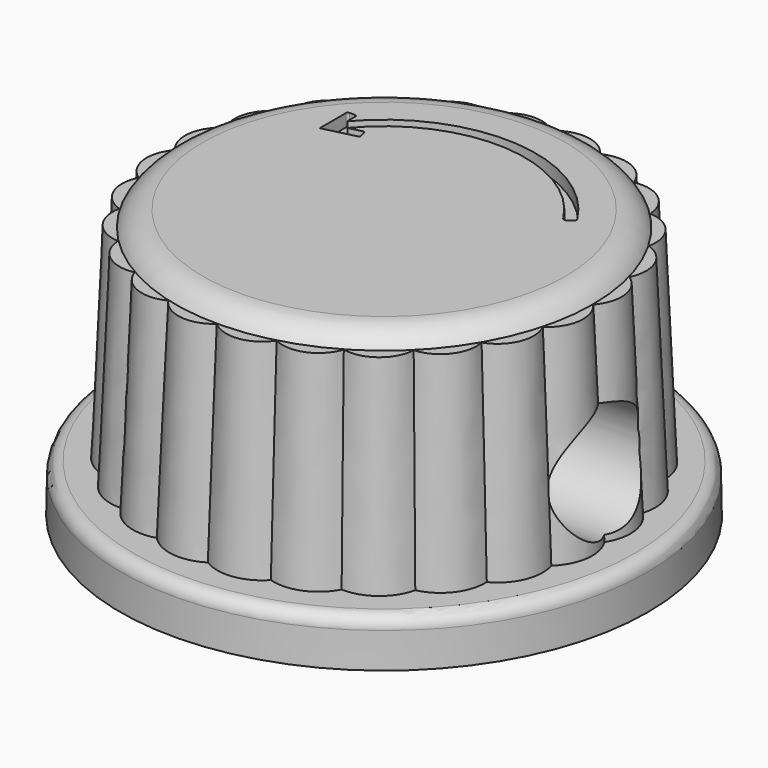
from build123d import *

# Parameters (mm, degrees)
F0_R                   = 8.35
F1_DEPTH               = 1.5
F1_TAPER               = 1
F2_R                   = 6.9
F3_DEPTH               = 6.5
F3_TAPER               = 2.5
F4_R                   = 6.6019829431
F5_DEPTH               = 0.5
F7_DEPTH               = 6.5
DRAFT_F7_DRAFTED_ANGLE = -2.5
F9_R                   = 0.4
F10_R                  = 3.9
F11_DEPTH              = 6.8
F12_R                  = 1.8
F13_DEPTH              = 25
F15_DEPTH              = 0.4


# Not quite as in the source:
# - a fillet or chamfer that OpenCascade refuses, or shapes differently, is made with other operations: its cross-section is extruded or revolved along the edge and cut away or added
# - an extrude with a draft is written as a straight extrude whose walls are then drafted


with BuildPart() as f1:
    # F0 (on Top) → F1 (new body)
    with BuildSketch(Plane.XY):
        Circle(F0_R)
    extrude(amount=F1_DEPTH, taper=F1_TAPER)

    # F2 (on face) → F3 (join)
    with BuildSketch(Plane.XY.offset(1.5)):
        Circle(F2_R)
    extrude(amount=F3_DEPTH, taper=F3_TAPER)

    # F4 (on face) → F5 (join)
    with BuildSketch(Plane.XY.offset(8)):
        Circle(F4_R)
    extrude(amount=F5_DEPTH)


with BuildPart() as f7_drafted:
    # F6 (on face) → F7 (new body, through all)
    with BuildSketch(Plane.XY.offset(8)):
        with BuildLine():
            ThreePointArc((6.3907621911, -1.7123995681), (6.8957390773, -0.9078412722), (6.6162038711, 0))
            ThreePointArc((6.6162038711, 0), (6.8957390773, 0.9078412722), (6.3907621911, 1.7123995681))
            ThreePointArc((6.3907621911, 1.7123995681), (6.4258058549, 2.6616559343), (5.729800629, 3.3081019355))
            ThreePointArc((5.729800629, 3.3081019355), (5.5179645827, 4.234083143), (4.678362623, 4.678362623))
            ThreePointArc((4.678362623, 4.678362623), (4.234083143, 5.5179645827), (3.3081019355, 5.729800629))
            ThreePointArc((3.3081019355, 5.729800629), (2.6616559343, 6.4258058549), (1.7123995681, 6.3907621911))
            ThreePointArc((1.7123995681, 6.3907621911), (0.9078412722, 6.8957390773), (0, 6.6162038711))
            ThreePointArc((0, 6.6162038711), (-0.9078412722, 6.8957390773), (-1.7123995681, 6.3907621911))
            ThreePointArc((-1.7123995681, 6.3907621911), (-2.6616559343, 6.4258058549), (-3.3081019355, 5.729800629))
            ThreePointArc((-3.3081019355, 5.729800629), (-4.234083143, 5.5179645827), (-4.678362623, 4.678362623))
            ThreePointArc((-4.678362623, 4.678362623), (-5.5179645827, 4.234083143), (-5.729800629, 3.3081019355))
            ThreePointArc((-5.729800629, 3.3081019355), (-6.4258058549, 2.6616559343), (-6.3907621911, 1.7123995681))
            ThreePointArc((-6.3907621911, 1.7123995681), (-6.8957390773, 0.9078412722), (-6.6162038711, 0))
            ThreePointArc((-6.6162038711, 0), (-6.8957390773, -0.9078412722), (-6.3907621911, -1.7123995681))
            ThreePointArc((-6.3907621911, -1.7123995681), (-6.4258058549, -2.6616559343), (-5.729800629, -3.3081019355))
            ThreePointArc((-5.729800629, -3.3081019355), (-5.5179645827, -4.234083143), (-4.678362623, -4.678362623))
            ThreePointArc((-4.678362623, -4.678362623), (-4.234083143, -5.5179645827), (-3.3081019355, -5.729800629))
            ThreePointArc((-3.3081019355, -5.729800629), (-2.6616559343, -6.4258058549), (-1.7123995681, -6.3907621911))
            ThreePointArc((-1.7123995681, -6.3907621911), (-0.9078412722, -6.8957390773), (0, -6.6162038711))
            ThreePointArc((0, -6.6162038711), (0.9078412722, -6.8957390773), (1.7123995681, -6.3907621911))
            ThreePointArc((1.7123995681, -6.3907621911), (2.6616559343, -6.4258058549), (3.3081019355, -5.729800629))
            ThreePointArc((3.3081019355, -5.729800629), (4.234083143, -5.5179645827), (4.678362623, -4.678362623))
            ThreePointArc((4.678362623, -4.678362623), (5.5179645827, -4.234083143), (5.729800629, -3.3081019355))
            ThreePointArc((5.729800629, -3.3081019355), (6.4258058549, -2.6616559343), (6.3907621911, -1.7123995681))
        make_face()
    extrude(amount=-F7_DEPTH)

    # draft_F7_drafted
    draft_f7_drafted_walls = [f7_drafted.faces().sort_by_distance(p)[0] for p in [
        (2.6616559343, -6.4258058549, 3.6666666667),
        (4.234083143, -5.5179645827, 3.6666666667),
        (5.5179645827, -4.234083143, 3.6666666667),
        (6.4258058549, -2.6616559343, 3.6666666667),
        (6.8957390773, -0.9078412722, 3.6666666667),
        (6.8957390773, 0.9078412722, 3.6666666667),
        (6.4258058549, 2.6616559343, 3.6666666667),
        (5.5179645827, 4.234083143, 3.6666666667),
        (4.234083143, 5.5179645827, 3.6666666667),
        (2.6616559343, 6.4258058549, 3.6666666667),
        (0.9078412722, 6.8957390773, 3.6666666667),
        (-0.9078412722, 6.8957390773, 3.6666666667),
        (-2.6616559343, 6.4258058549, 3.6666666667),
        (-4.234083143, 5.5179645827, 3.6666666667),
        (-5.5179645827, 4.234083143, 3.6666666667),
        (-6.4258058549, 2.6616559343, 3.6666666667),
        (-6.8957390773, 0.9078412722, 3.6666666667),
        (-6.8957390773, -0.9078412722, 3.6666666667),
        (-6.4258058549, -2.6616559343, 3.6666666667),
        (-5.5179645827, -4.234083143, 3.6666666667),
        (-4.234083143, -5.5179645827, 3.6666666667),
        (-2.6616559343, -6.4258058549, 3.6666666667),
        (-0.9078412722, -6.8957390773, 3.6666666667),
        (0.9078412722, -6.8957390773, 3.6666666667),
    ]]
    draft(draft_f7_drafted_walls, neutral_plane=Plane(origin=(0, 0, 8), x_dir=(1, 0, 0), z_dir=(0, 0, -1)), angle=DRAFT_F7_DRAFTED_ANGLE)


with BuildPart() as f1_1:
    add(f1.part)

    # join_F7_drafted: union F7_drafted
    add(f7_drafted.part)

    # F8: fillet of radius 1 on 1 edges, made by hand

    # F8_s1 → F8_t2 (revolve, cut)
    with BuildSketch(Plane.XZ):
        with BuildLine():
            ThreePointArc((6.6019829431, 8), (6.2359575393, 8.3660254038), (5.7359575393, 8.5))
            Line((5.7359575393, 8.5), (6.6019829431, 8.5))
            Line((6.6019829431, 8.5), (6.6019829431, 8))
        make_face()
    revolve(axis=Axis((0, 0, 8.5), (0, 0, 1)), mode=Mode.SUBTRACT)

    # F9
    f9_edges = [f1_1.edges().sort_by_distance(p)[0] for p in [
        (-8.323817, 0, 1.5),
    ]]
    fillet(f9_edges, radius=F9_R)

    # F10 (on face) → F11 (cut)
    with BuildSketch(Plane(origin=(0, 0, 0), x_dir=(1, 0, 0), z_dir=(0, 0, -1))):
        Circle(F10_R)
    extrude(amount=-F11_DEPTH, mode=Mode.SUBTRACT)

    # F12 (on Right) → F13 (cut)
    with BuildSketch(Plane.YZ):
        with Locations((0, 3.5)):
            Circle(F12_R)
    extrude(amount=F13_DEPTH, mode=Mode.SUBTRACT)

    # F14 (on face) → F15 (cut)
    with BuildSketch(Plane.XY.offset(8.5)):
        with BuildLine():
            ThreePointArc((4.0182745738, 2.4358713944), (4.0638071122, 2.4986082213), (4.0508280388, 2.5750324659))
            ThreePointArc((4.0508280388, 2.5750324659), (0.3332787647, 4.7884157364), (-3.6550484848, 3.1113695657))
            Line((-3.6550484848, 3.1113695657), (-3.6550484848, 2.7795751277))
            Line((-3.6550484848, 2.7795751277), (-3.430580727, 2.8343633986))
            ThreePointArc((-3.430580727, 2.8343633986), (0.2747733656, 4.4415087074), (3.7537793514, 2.3899038853))
            ThreePointArc((3.7537793514, 2.3899038853), (3.8153903675, 2.3462302819), (3.8899727294, 2.3580950287))
            Line((3.8899727294, 2.3580950287), (4.0182745738, 2.4358713944))
        make_face()
        with BuildLine():
            Line((-3.6550484848, 2.7795751277), (-3.6550484848, 3.1113695657))
            ThreePointArc((-3.6550484848, 3.1113695657), (-3.8100807859, 2.9194664589), (-3.9550484848, 2.7198513715))
            Line((-3.9550484848, 2.7198513715), (-3.9550484848, 2.3975438439))
            Line((-3.9550484848, 2.3975438439), (-3.7099685017, 2.4573631633))
            ThreePointArc((-3.7099685017, 2.4573631633), (-3.5752472805, 2.6495484301), (-3.430580727, 2.8343633986))
            Line((-3.430580727, 2.8343633986), (-3.6550484848, 2.7795751277))
        make_face()
        with BuildLine():
            ThreePointArc((-3.9550484848, 2.7198513715), (-3.8100807859, 2.9194664589), (-3.6550484848, 3.1113695657))
            Line((-3.6550484848, 3.1113695657), (-3.6550484848, 3.4375438439))
            ThreePointArc((-3.6550484848, 3.4375438439), (-3.6726220779, 3.4799702507), (-3.7150484848, 3.4975438439))
            Line((-3.7150484848, 3.4975438439), (-3.8950484848, 3.4975438439))
            ThreePointArc((-3.8950484848, 3.4975438439), (-3.9374748916, 3.4799702507), (-3.9550484848, 3.4375438439))
            Line((-3.9550484848, 3.4375438439), (-3.9550484848, 2.7198513715))
        make_face()
        with BuildLine():
            Line((-3.0158447502, 2.9355924894), (-3.430580727, 2.8343633986))
            ThreePointArc((-3.430580727, 2.8343633986), (-3.5752472805, 2.6495484301), (-3.7099685017, 2.4573631633))
            Line((-3.7099685017, 2.4573631633), (-2.9447088324, 2.6441483589))
            ThreePointArc((-2.9447088324, 2.6441483589), (-2.9076594538, 2.6712808988), (-2.9006471899, 2.7166643686))
            Line((-2.9006471899, 2.7166643686), (-2.9433287405, 2.8915308469))
            ThreePointArc((-2.9433287405, 2.8915308469), (-2.9704612804, 2.9285802255), (-3.0158447502, 2.9355924894))
        make_face()
    extrude(amount=-F15_DEPTH, mode=Mode.SUBTRACT)


solid = f1_1.part
